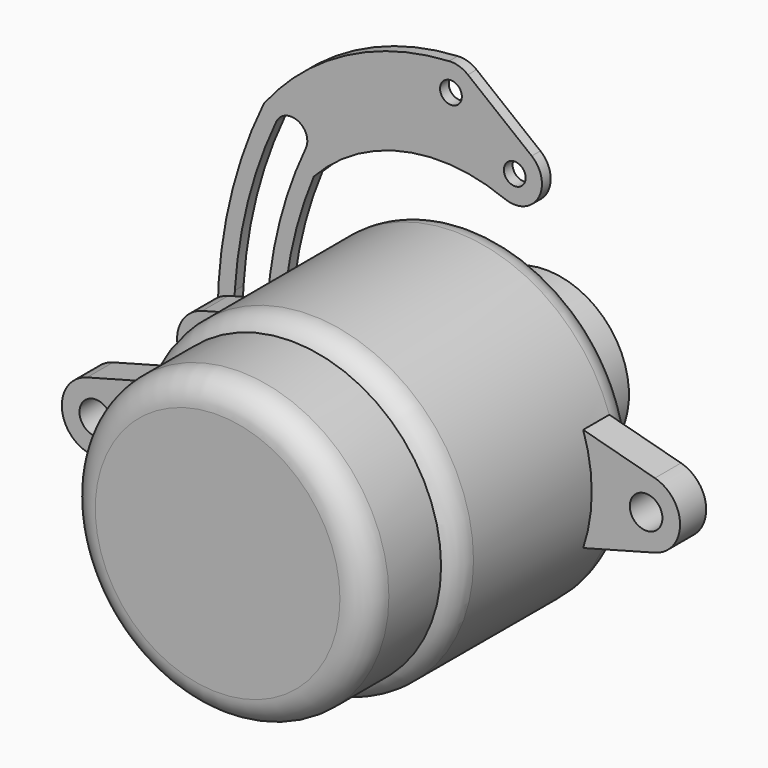
from build123d import *

# Parameters (mm, degrees)
F0_R      = 60
F1_DEPTH  = 85
F2_R      = 55
F3_DEPTH  = 34
F5_R      = 6
F6_DEPTH  = 12
F7_R      = 30.5
F8_DEPTH  = 20
F10_R     = 6
F11_DEPTH = 12
F13_R     = 6
F14_DEPTH = 12
F15_R     = 4
F16_DEPTH = 4


# Not quite as in the source:
# - a fillet or chamfer that OpenCascade refuses, or shapes differently, is made with other operations: its cross-section is extruded or revolved along the edge and cut away or added


with BuildPart() as f1:
    # F0 (on Front) → F1 (new body)
    with BuildSketch(Plane.XZ):
        Circle(F0_R)
    extrude(amount=F1_DEPTH)

    # F2 (on face) → F3 (join)
    with BuildSketch(Plane.XZ.offset(85)):
        Circle(F2_R)
    extrude(amount=F3_DEPTH)

    # F4: fillet of radius 10 on 3 edges, made by hand

    # F4_s1 → F4_t2 (revolve, cut)
    with BuildSketch(Plane.XY):
        with BuildLine():
            ThreePointArc((60, -10), (57.0710678119, -2.9289321881), (50, 0))
            Line((50, 0), (60, 0))
            Line((60, 0), (60, -10))
        make_face()
    revolve(axis=Axis((0, 0, 0), (0, -1, 0)), mode=Mode.SUBTRACT)

    # F4_s3 → F4_t4 (revolve, cut)
    with BuildSketch(Plane.XY):
        with BuildLine():
            ThreePointArc((60, -76.3397459622), (58.6602540378, -81.3397459622), (55, -85))
            Line((55, -85), (60, -85))
            Line((60, -85), (60, -76.3397459622))
        make_face()
    revolve(axis=Axis((0, -85, 0), (0, -1, 0)), mode=Mode.SUBTRACT)

    # F4_s5 → F4_t6 (revolve, cut)
    with BuildSketch(Plane.XY):
        with BuildLine():
            ThreePointArc((55, -109), (52.0710678119, -116.0710678119), (45, -119))
            Line((45, -119), (55, -119))
            Line((55, -119), (55, -109))
        make_face()
    revolve(axis=Axis((0, -119, 0), (0, -1, 0)), mode=Mode.SUBTRACT)

    # F5 (on face) → F6 (join)
    with BuildSketch(Plane(origin=(0, 0, 0), x_dir=(-1, 0, 0), z_dir=(0, 1, 0))):
        Circle(F5_R)
    extrude(amount=F6_DEPTH)

    # F7 (on face) → F8 (join)
    with BuildSketch(Plane(origin=(0, 12, 0), x_dir=(-1, 0, 0), z_dir=(0, 1, 0))):
        Circle(F7_R)
    extrude(amount=F8_DEPTH)

    # F10 (on offset) → F11 (join)
    with BuildSketch(Plane.XZ.offset(10)):
        with BuildLine():
            Line((56.8653269235, -19.1398692231), (83.2352380638, -12.0740728286))
            ThreePointArc((83.2352380638, -12.0740728286), (92.5, 0), (83.2352380638, 12.0740728286))
            Line((83.2352380638, 12.0740728286), (56.8653269235, 19.1398692231))
            ThreePointArc((56.8653269235, 19.1398692231), (60, 0), (56.8653269235, -19.1398692231))
        make_face()
        with Locations((80, 0)):
            Circle(F10_R, mode=Mode.SUBTRACT)
        with BuildLine():
            Line((-56.8653269235, 19.1398692231), (-83.2352380638, 12.0740728286))
            ThreePointArc((-83.2352380638, 12.0740728286), (-92.5, 0), (-83.2352380638, -12.0740728286))
            Line((-83.2352380638, -12.0740728286), (-56.8653269235, -19.1398692231))
            ThreePointArc((-56.8653269235, -19.1398692231), (-60, 0), (-56.8653269235, 19.1398692231))
        make_face()
        with Locations((-80, 0)):
            Circle(F10_R, mode=Mode.SUBTRACT)
    extrude(amount=F11_DEPTH)

    # F13 (on offset) → F14 (join)
    with BuildSketch(Plane.XZ.offset(75)):
        with BuildLine():
            Line((-83.2352380638, -12.0740728286), (-56.8653269235, -19.1398692231))
            ThreePointArc((-56.8653269235, -19.1398692231), (-60, 0), (-56.8653269235, 19.1398692231))
            Line((-56.8653269235, 19.1398692231), (-83.2352380638, 12.0740728286))
            ThreePointArc((-83.2352380638, 12.0740728286), (-92.5, 0), (-83.2352380638, -12.0740728286))
        make_face()
        with Locations((-80, 0)):
            Circle(F13_R, mode=Mode.SUBTRACT)
    extrude(amount=-F14_DEPTH)


with BuildPart() as f16:
    # F15 (on Front) → F16 (new body)
    with BuildSketch(Plane.XZ):
        with BuildLine():
            ThreePointArc((-74, -1.341e-07), (-80.000000067, -6), (-86, 0))
            ThreePointArc((-86, 0), (-85.9156035459, 5.2926836293), (-85.6625, 10.5799855269))
            ThreePointArc((-85.6625, 10.5799855269), (-90.2944159621, 6.1664414373), (-92, 0))
            ThreePointArc((-92, 0), (-80, -12), (-68, 0))
            ThreePointArc((-68, 0), (-69.5107197578, 5.8288077683), (-73.6625, 10.1899996933))
            ThreePointArc((-73.6625, 10.1899996933), (-73.9156018755, 5.0977935734), (-74, -1.341e-07))
        make_face()
        with BuildLine():
            ThreePointArc((-92, 0), (-90.2944159621, 6.1664414373), (-85.6625, 10.5799855269))
            ThreePointArc((-85.6625, 10.5799855269), (-80.8371948593, 41.077935072), (-70.4470926481, 70.154631449))
            ThreePointArc((-70.4470926481, 70.154631449), (-62.4735363554, 73.0567686007), (-59.5713992036, 65.0832123081))
            ThreePointArc((-59.5713992036, 65.0832123081), (-69.1638230548, 38.2903890247), (-73.6625, 10.1899996933))
            ThreePointArc((-73.6625, 10.1899996933), (-69.5107197578, 5.8288077683), (-68, 0))
            ThreePointArc((-68, 0), (-65.1226661747, 29.0415523406), (-56.602543752, 56.9538852096))
            ThreePointArc((-56.602543752, 56.9538852096), (-23.9720972385, 75.7077221411), (13.5313898709, 72.5548038174))
            ThreePointArc((13.5313898709, 72.5548038174), (25.933712547, 76.7674690687), (23.5271965971, 89.6427491536))
            Line((23.5271965971, 89.6427491536), (0.0489518915, 108.3181882527))
            ThreePointArc((0.0489518915, 108.3181882527), (-3.2091779587, 110.0418089305), (-6.8704149318, 110.4679804784))
            ThreePointArc((-6.8704149318, 110.4679804784), (-44.8441817754, 99.9525565554), (-74.9901091983, 74.5792601914))
            ThreePointArc((-74.9901091983, 74.5792601914), (-87.6936176217, 38.247230082), (-92, 0))
        make_face()
        with Locations((-6.1761944749, 100.4921066842)):
            Circle(F15_R, mode=Mode.SUBTRACT)
        with Locations((17.3020502307, 81.8166675851)):
            Circle(F15_R, mode=Mode.SUBTRACT)
    extrude(amount=F16_DEPTH)


solid = Compound([f1.part, f16.part])
